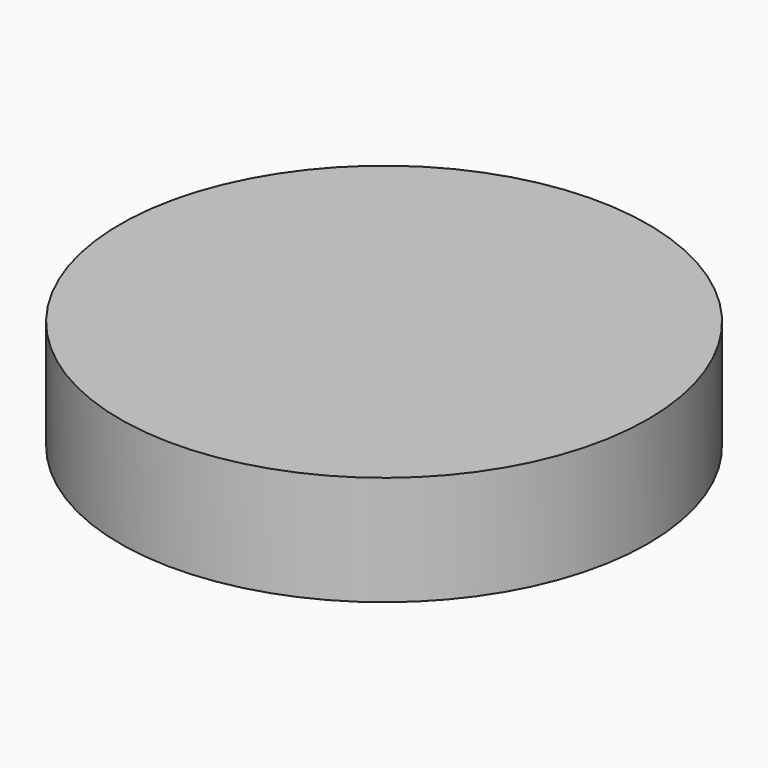
from build123d import *

# Parameters (mm, degrees)
F0_W = 72.6498719305
F0_H = 30.1429410465


# Not quite as in the source:
# - the program builds the solid bodies; features that only make, move or delete a surface that nothing else refers to are left out


with BuildPart() as f1:
    # F0 (on Front) → F1 (revolve)
    with BuildSketch(Plane.XZ):
        with Locations((-11.7273898795, 19.3971504923)):
            Rectangle(F0_W, F0_H)
    revolve(axis=Axis((-48.0523258448, 0, 19.3971504923), (0, 0, -1)))


solid = f1.part
